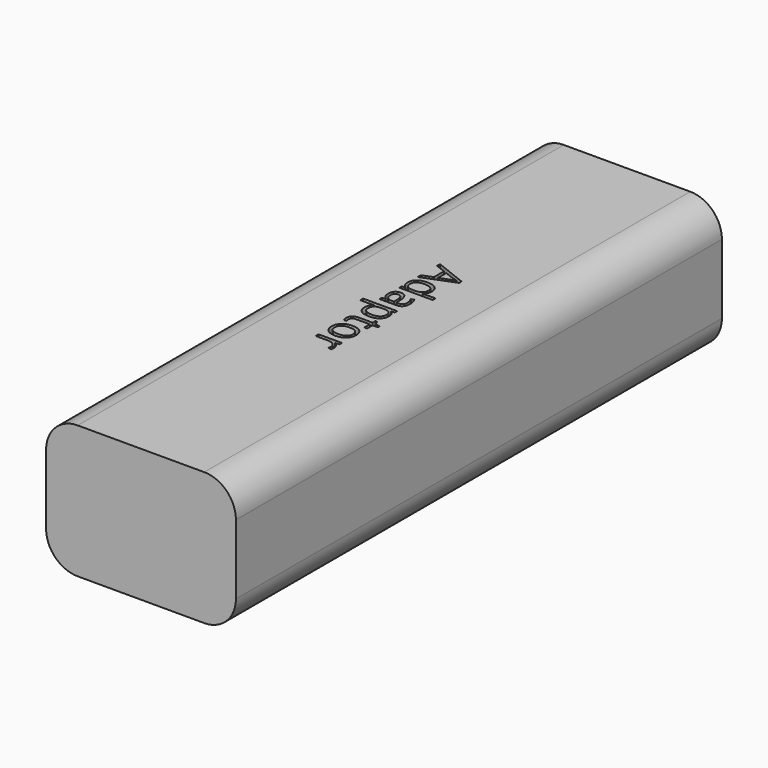
from build123d import *

# Parameters (mm, degrees)
F0_W         = 30
F0_H         = 96
F1_DEPTH     = 21
F2_R         = 5
F3_W         = 16
F3_H         = 13
F4_DEPTH     = 25
F6_TEXT_SIZE = 6.9444444444
F7_DEPTH     = 1
F9_W         = 12.5
F9_H         = 5
F10_DEPTH    = 5


# Not quite as in the source:
# - Text() gives the source's letters only with a copy of the font that has no kerning and outlines rounded to 1/6400 em; it was checked with that copy


with BuildPart() as f1:
    # F0 (on Top) → F1 (new body)
    with BuildSketch(Plane.XY):
        Rectangle(F0_W, F0_H)
    extrude(amount=F1_DEPTH)

    # F2
    f2_edges = [f1.edges().sort_by_distance(p)[0] for p in [
        (15, 0, 21),
        (-15, 0, 21),
        (15, 0, 0),
        (-15, 0, 0),
    ]]
    fillet(f2_edges, radius=F2_R)

    # F3 (on face) → F4 (cut)
    with BuildSketch(Plane(origin=(0, 48, 0), x_dir=(-1, 0, 0), z_dir=(0, 1, 0))):
        with Locations((0, 9.5)):
            Rectangle(F3_W, F3_H)
    extrude(amount=-F4_DEPTH, mode=Mode.SUBTRACT)

    # F6 (on offset) → F7 (cut)
    with BuildSketch(Plane.XY.offset(21)):
        with Locations(Location((-2.0111614147, 13.5827610655), (0, 0, -90))):
            Text('Adaptor', F6_TEXT_SIZE, font='Open Sans', text_align=(TextAlign.LEFT, TextAlign.BOTTOM))
    extrude(amount=-F7_DEPTH, mode=Mode.SUBTRACT)

    # F9 (on offset) → F10 (cut)
    with BuildSketch(Plane(origin=(0, 0, 0), x_dir=(1, 0, 0), z_dir=(0, 0, -1))):
        with Locations((0, 21.5)):
            Rectangle(F9_W, F9_H)
        with Locations((0, 5.5)):
            Rectangle(F9_W, F9_H)
        with Locations((0, -10.5)):
            Rectangle(F9_W, F9_H)
    extrude(amount=-F10_DEPTH, mode=Mode.SUBTRACT)


solid = f1.part
